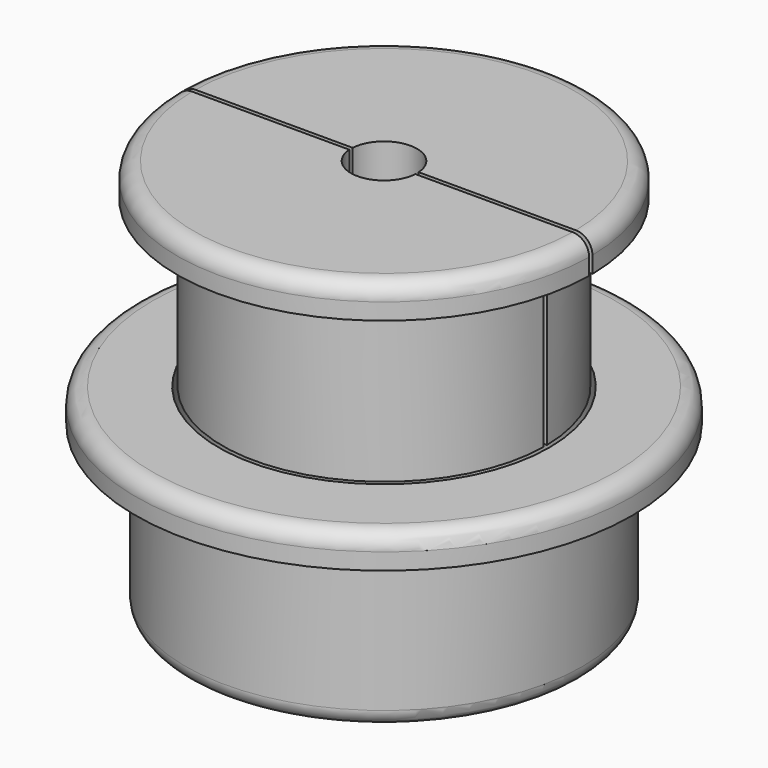
from build123d import *

# Parameters (mm, degrees)
F2_R     = 0.99999
F3_R     = 9.75
F3_R_2   = 2
F4_DEPTH = 10
F5_R     = 12.5
F5_R_2   = 2
F6_DEPTH = 2
F7_R     = 1
F8_W     = 25
F8_H     = 0.25
F9_DEPTH = 12


# Not quite as in the source:
# - a fillet or chamfer is up to 0.001 mm smaller than in the source, because OpenCascade refuses the exact size
# - a feature names something its author has since deleted; it is built from what else it names


with BuildPart() as f1:
    # F0 (on Front) → F1 (revolve)
    with BuildSketch(Plane.XZ):
        Polygon((10, 12), (10, 0), (12, 0), (12, 10), (15, 10), (15, 12), align=None)
    revolve(axis=Axis((0, 0, 14.2161818221), (0, 0, 1)))

    # F2 (radius 1 in the source; OpenCascade refuses exactly that, so slightly less here)
    f2_edges = [f1.edges().sort_by_distance(p)[0] for p in [
        (-10, 0, 0),
        (-12, 0, 0),
        (-15, 0, 12),
    ]]
    fillet(f2_edges, radius=F2_R)


with BuildPart() as f4:
    # F3 (on face) → F4 (new body)
    with BuildSketch(Plane.XY.offset(12)):
        Circle(F3_R)
        Circle(F3_R_2, mode=Mode.SUBTRACT)
    extrude(amount=F4_DEPTH)

    # F5 (on face) → F6 (join)
    with BuildSketch(Plane.XY.offset(22)):
        Circle(F5_R)
        Circle(F5_R_2, mode=Mode.SUBTRACT)
    extrude(amount=F6_DEPTH)

    # F7
    f7_edges = [f4.edges().sort_by_distance(p)[0] for p in [
        (-12.5, 0, 24),
    ]]
    fillet(f7_edges, radius=F7_R)

    # F8 (on face) → F9 (cut, through all)
    with BuildSketch(Plane.XY.offset(24)):
        Rectangle(F8_W, F8_H)
    extrude(amount=-F9_DEPTH, mode=Mode.SUBTRACT)


solid = Compound([f1.part, f4.part])
